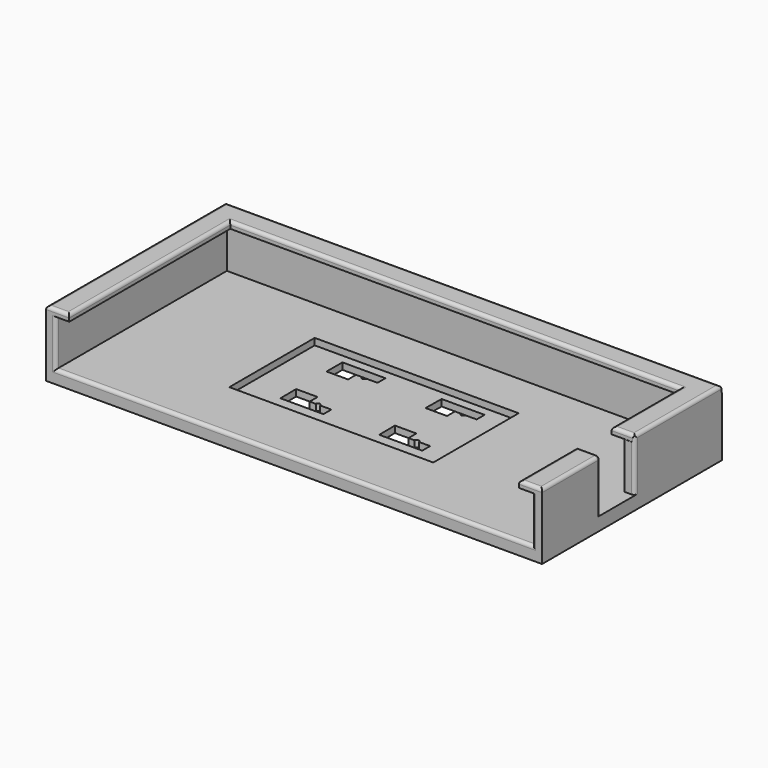
from build123d import *

# Parameters (mm, degrees)
F0_W         = 150
F0_H         = 68
F0_W_2       = 61.6867046999
F0_H_2       = 32.2795761846
F1_DEPTH     = 2
F2_W         = 3
F2_H         = 3.4045838118
F2_W_2       = 144
F2_H_2       = 64.5954161882
F2_H_3       = 29.5954161882
F2_H_4       = 22
F3_DEPTH     = 14
F4_W         = 4.8811412584
F4_H         = 7
F4_W_2       = 136
F4_W_3       = 7
F4_H_2       = 25.8289493918
F4_H_3       = 22
F5_DEPTH     = 2
F6_T1_DEPTH  = 72.8877383471
F6_T3_DEPTH  = 12
F6_T5_DEPTH  = 63.3877383471
F6_T7_DEPTH  = 136
F6_T9_DEPTH  = 28.3289493918
F6_T11_DEPTH = 12
F6_T13_DEPTH = 37.8289493918
F6_T15_DEPTH = 155
F6_T17_DEPTH = 23.5
F6_T19_DEPTH = 8.5
F6_T21_DEPTH = 27
F6_T23_DEPTH = 144
F6_T25_DEPTH = 14
F6_T27_DEPTH = 15
F6_T29_DEPTH = 16.5
F6_S33_W     = 1
F6_S33_H     = 1
F6_T34_DEPTH = 1
F6_T41_DEPTH = 65.8877383471
F6_T45_DEPTH = 138.5
F6_T52_DEPTH = 138.5
F6_T56_DEPTH = 30.8289493918
F6_T63_DEPTH = 146.5
F6_T67_DEPTH = 16.5
F6_T74_DEPTH = 146.5
F6_T78_DEPTH = 16.5
F7_W         = 150
F7_H         = 68
F7_W_2       = 61.6867046999
F7_H_2       = 32.2795761846
F8_DEPTH     = 2
F9_W         = 73.8973718075
F9_H         = 39.0960725045
F9_W_2       = 61.6867046999
F9_H_2       = 32.2795761846
F10_DEPTH    = 2


# Not quite as in the source:
# - a fillet or chamfer that OpenCascade refuses, or shapes differently, is made with other operations: its cross-section is extruded or revolved along the edge and cut away or added
# - a feature names something its author has since deleted; it is built from what else it names


with BuildPart() as f1:
    # F0 (on Top) → F1 (new body)
    with BuildSketch(Plane.XY):
        with Locations((75, 34)):
            Rectangle(F0_W, F0_H)
        with Locations((71.4499814534, 34.6545311671)):
            Rectangle(F0_W_2, F0_H_2, mode=Mode.SUBTRACT)
    extrude(amount=F1_DEPTH)

    # F2 (on face) → F3 (join)
    with BuildSketch(Plane.XY.offset(2)):
        with Locations((1.5, 66.2977080941)):
            Rectangle(F2_W, F2_H)
        with Locations((75, 66.2977080941)):
            Rectangle(F2_W_2, F2_H)
        with Locations((1.5, 32.2977080941)):
            Rectangle(F2_W, F2_H_2)
        with Locations((148.5, 66.2977080941)):
            Rectangle(F2_W, F2_H)
        with Locations((148.5, 49.7977080941)):
            Rectangle(F2_W, F2_H_3)
        with Locations((148.5, 11)):
            Rectangle(F2_W, F2_H_4)
    extrude(amount=F3_DEPTH)

    # F4 (on face) → F5 (join)
    with BuildSketch(Plane.XY.offset(16)):
        Polygon((0, 67.8877383471), (0, 0), (7, 0), (7, 60.8877383471), (2.1188587416, 60.8877383471), (2.1188587416, 67.8877383471), align=None)
        with Locations((4.5594293708, 64.3877383471)):
            Rectangle(F4_W, F4_H)
        with Locations((75, 64.3877383471)):
            Rectangle(F4_W_2, F4_H)
        with Locations((146.5, 64.3877383471)):
            Rectangle(F4_W_3, F4_H)
        with Locations((146.5, 47.9732636511)):
            Rectangle(F4_W_3, F4_H_2)
        with Locations((146.5, 11)):
            Rectangle(F4_W_3, F4_H_3)
    extrude(amount=F5_DEPTH)

    # F6: fillet of radius 1 on 17 edges, made by hand

    # F6_s2 → F6_t1 (cut)
    with BuildSketch(Plane.XZ.offset(-70.3877383471)):
        with BuildLine():
            ThreePointArc((0, 17), (0.2928932188, 17.7071067812), (1, 18))
            Line((1, 18), (0, 18))
            Line((0, 18), (0, 17))
        make_face()
    extrude(amount=F6_T1_DEPTH, mode=Mode.SUBTRACT)

    # F6_s4 → F6_t3 (cut)
    with BuildSketch(Plane.YZ.offset(-2.5)):
        with BuildLine():
            ThreePointArc((0, 17), (0.2928932188, 17.7071067812), (1, 18))
            Line((1, 18), (0, 18))
            Line((0, 18), (0, 17))
        make_face()
    extrude(amount=F6_T3_DEPTH, mode=Mode.SUBTRACT)

    # F6_s6 → F6_t5 (cut)
    with BuildSketch(Plane.XZ.offset(-60.8877383471)):
        with BuildLine():
            ThreePointArc((7, 17), (6.7071067812, 17.7071067812), (6, 18))
            Line((6, 18), (7, 18))
            Line((7, 18), (7, 17))
        make_face()
    extrude(amount=F6_T5_DEPTH, mode=Mode.SUBTRACT)

    # F6_s8 → F6_t7 (cut)
    with BuildSketch(Plane.YZ.offset(7)):
        with BuildLine():
            ThreePointArc((60.8877383471, 17), (61.1806315659, 17.7071067812), (61.8877383471, 18))
            Line((61.8877383471, 18), (60.8877383471, 18))
            Line((60.8877383471, 18), (60.8877383471, 17))
        make_face()
    extrude(amount=F6_T7_DEPTH, mode=Mode.SUBTRACT)

    # F6_s10 → F6_t9 (cut)
    with BuildSketch(Plane.XZ.offset(-60.8877383471)):
        with BuildLine():
            ThreePointArc((143, 17), (143.2928932188, 17.7071067812), (144, 18))
            Line((144, 18), (143, 18))
            Line((143, 18), (143, 17))
        make_face()
    extrude(amount=F6_T9_DEPTH, mode=Mode.SUBTRACT)

    # F6_s12 → F6_t11 (cut)
    with BuildSketch(Plane.YZ.offset(140.5)):
        with BuildLine():
            ThreePointArc((35.0587889552, 17), (35.351682174, 17.7071067812), (36.0587889552, 18))
            Line((36.0587889552, 18), (35.0587889552, 18))
            Line((35.0587889552, 18), (35.0587889552, 17))
        make_face()
        with BuildLine():
            ThreePointArc((1, 18), (0.2928932188, 17.7071067812), (0, 17))
            Line((0, 17), (0, 18))
            Line((0, 18), (1, 18))
        make_face()
    extrude(amount=F6_T11_DEPTH, mode=Mode.SUBTRACT)

    # F6_s14 → F6_t13 (cut)
    with BuildSketch(Plane.XZ.offset(-70.3877383471)):
        with BuildLine():
            ThreePointArc((150, 17), (149.7071067812, 17.7071067812), (149, 18))
            Line((149, 18), (150, 18))
            Line((150, 18), (150, 17))
        make_face()
    extrude(amount=F6_T13_DEPTH, mode=Mode.SUBTRACT)

    # F6_s16 → F6_t15 (cut)
    with BuildSketch(Plane.YZ.offset(-2.5)):
        with BuildLine():
            ThreePointArc((66.8877383471, 18), (67.5948451282, 17.7071067812), (67.8877383471, 17))
            Line((67.8877383471, 17), (67.8877383471, 18))
            Line((67.8877383471, 18), (66.8877383471, 18))
        make_face()
    extrude(amount=F6_T15_DEPTH, mode=Mode.SUBTRACT)

    # F6_s18 → F6_t17 (cut)
    with BuildSketch(Plane.XZ.offset(-21)):
        with BuildLine():
            ThreePointArc((149, 18), (149.7071067812, 17.7071067812), (150, 17))
            Line((150, 17), (150, 18))
            Line((150, 18), (149, 18))
        make_face()
    extrude(amount=F6_T17_DEPTH, mode=Mode.SUBTRACT)

    # F6_s20 → F6_t19 (cut)
    with BuildSketch(Plane.YZ.offset(140.5)):
        with BuildLine():
            ThreePointArc((21, 18), (21.7071067812, 17.7071067812), (22, 17))
            Line((22, 17), (22, 18))
            Line((22, 18), (21, 18))
        make_face()
    extrude(amount=F6_T19_DEPTH, mode=Mode.SUBTRACT)

    # F6_s22 → F6_t21 (cut)
    with BuildSketch(Plane.XZ.offset(-24.5)):
        with BuildLine():
            ThreePointArc((143, 17), (143.2928932188, 17.7071067812), (144, 18))
            Line((144, 18), (143, 18))
            Line((143, 18), (143, 17))
        make_face()
    extrude(amount=F6_T21_DEPTH, mode=Mode.SUBTRACT)

    # F6_s24 → F6_t23 (cut)
    with BuildSketch(Plane.YZ.offset(3)):
        with BuildLine():
            ThreePointArc((1, 2), (0.2928932188, 1.7071067812), (0, 1))
            Line((0, 1), (0, 2))
            Line((0, 2), (1, 2))
        make_face()
    extrude(amount=F6_T23_DEPTH, mode=Mode.SUBTRACT)

    # F6_s26 → F6_t25 (cut)
    with BuildSketch(Plane.XY.offset(2)):
        with BuildLine():
            ThreePointArc((3, 1), (2.7071067812, 0.2928932188), (2, 0))
            Line((2, 0), (3, 0))
            Line((3, 0), (3, 1))
        make_face()
        with BuildLine():
            ThreePointArc((147, 1), (147.2928932188, 0.2928932188), (148, 0))
            Line((148, 0), (147, 0))
            Line((147, 0), (147, 1))
        make_face()
    extrude(amount=F6_T25_DEPTH, mode=Mode.SUBTRACT)

    # F6_s28 → F6_t27 (cut)
    with BuildSketch(Plane.XY.offset(2)):
        with BuildLine():
            ThreePointArc((149, 22), (149.7071067812, 21.7071067812), (150, 21))
            Line((150, 21), (150, 22))
            Line((150, 22), (149, 22))
        make_face()
    extrude(amount=F6_T27_DEPTH, mode=Mode.SUBTRACT)

    # F6_s30 → F6_t29 (cut)
    with BuildSketch(Plane.XY.offset(2)):
        with BuildLine():
            ThreePointArc((149, 35), (149.7071067812, 35.2928932188), (150, 36))
            Line((150, 36), (150, 35))
            Line((150, 35), (149, 35))
        make_face()
    extrude(amount=F6_T29_DEPTH, mode=Mode.SUBTRACT)


with BuildPart() as f6_tool32:
    # F6_s33 → F6_t34 (new body)
    with BuildSketch(Plane.XZ.offset(-21)):
        with Locations((149.5, 17.5)):
            Rectangle(F6_S33_W, F6_S33_H)
    extrude(amount=-F6_T34_DEPTH)

    # F6_s35 → F6_t36 (revolve, cut)
    with BuildSketch(Plane(origin=(149, 21, 17), x_dir=(-0.7071067812, 0, -0.7071067812), z_dir=(0.7071067812, 0, -0.7071067812))):
        with BuildLine():
            ThreePointArc((0, -1), (1, 0), (0, 1))
            Line((0, 1), (0, -1))
        make_face()
    revolve(axis=Axis((149, 21, 17), (0, 1, 0)), mode=Mode.SUBTRACT)


with BuildPart() as f1_1:
    add(f1.part)

    # F6_t31: cut F6_tool32
    add(f6_tool32.part, mode=Mode.SUBTRACT)


with BuildPart() as f6_tool39:
    # F6_s40 → F6_t41 (new body)
    with BuildSketch(Plane.XZ.offset(2.5)):
        with BuildLine():
            ThreePointArc((7, 17), (6.7071067812, 17.7071067812), (6, 18))
            Line((6, 18), (7, 18))
            Line((7, 18), (7, 17))
        make_face()
    extrude(amount=-F6_T41_DEPTH)

    split(bisect_by=Plane.XZ.offset(-60.8877383471), keep=Keep.BOTTOM)


with BuildPart() as f6_tool43:
    # F6_s44 → F6_t45 (new body)
    with BuildSketch(Plane.YZ.offset(4.5)):
        with BuildLine():
            ThreePointArc((60.8877383471, 17), (61.1806315659, 17.7071067812), (61.8877383471, 18))
            Line((61.8877383471, 18), (60.8877383471, 18))
            Line((60.8877383471, 18), (60.8877383471, 17))
        make_face()
    extrude(amount=F6_T45_DEPTH)

    split(bisect_by=Plane.YZ.offset(7), keep=Keep.BOTTOM)


with BuildPart() as f6_tool39_1:
    add(f6_tool39.part)

    # F6_t47: intersect F6_tool43
    add(f6_tool43.part, mode=Mode.INTERSECT)


with BuildPart() as f1_2:
    add(f1_1.part)

    # F6_t37: cut F6_tool39
    add(f6_tool39_1.part, mode=Mode.SUBTRACT)


with BuildPart() as f6_tool50:
    # F6_s51 → F6_t52 (new body)
    with BuildSketch(Plane.YZ.offset(7)):
        with BuildLine():
            ThreePointArc((60.8877383471, 17), (61.1806315659, 17.7071067812), (61.8877383471, 18))
            Line((61.8877383471, 18), (60.8877383471, 18))
            Line((60.8877383471, 18), (60.8877383471, 17))
        make_face()
    extrude(amount=F6_T52_DEPTH)

    split(bisect_by=Plane.YZ.offset(143), keep=Keep.TOP)


with BuildPart() as f6_tool54:
    # F6_s55 → F6_t56 (new body)
    with BuildSketch(Plane.XZ.offset(-63.3877383471)):
        with BuildLine():
            ThreePointArc((143, 17), (143.2928932188, 17.7071067812), (144, 18))
            Line((144, 18), (143, 18))
            Line((143, 18), (143, 17))
        make_face()
    extrude(amount=F6_T56_DEPTH)

    split(bisect_by=Plane.XZ.offset(-60.8877383471), keep=Keep.BOTTOM)


with BuildPart() as f6_tool50_1:
    add(f6_tool50.part)

    # F6_t58: intersect F6_tool54
    add(f6_tool54.part, mode=Mode.INTERSECT)


with BuildPart() as f1_3:
    add(f1_2.part)

    # F6_t48: cut F6_tool50
    add(f6_tool50_1.part, mode=Mode.SUBTRACT)


with BuildPart() as f6_tool61:
    # F6_s62 → F6_t63 (new body)
    with BuildSketch(Plane.YZ.offset(0.5)):
        with BuildLine():
            ThreePointArc((1, 2), (0.2928932188, 1.7071067812), (0, 1))
            Line((0, 1), (0, 2))
            Line((0, 2), (1, 2))
        make_face()
    extrude(amount=F6_T63_DEPTH)

    split(bisect_by=Plane.YZ.offset(3), keep=Keep.BOTTOM)


with BuildPart() as f6_tool65:
    # F6_s66 → F6_t67 (new body)
    with BuildSketch(Plane.XY.offset(-0.5)):
        with BuildLine():
            ThreePointArc((3, 1), (2.7071067812, 0.2928932188), (2, 0))
            Line((2, 0), (3, 0))
            Line((3, 0), (3, 1))
        make_face()
    extrude(amount=F6_T67_DEPTH)

    split(bisect_by=Plane.XY.offset(2), keep=Keep.BOTTOM)


with BuildPart() as f6_tool61_1:
    add(f6_tool61.part)

    # F6_t69: intersect F6_tool65
    add(f6_tool65.part, mode=Mode.INTERSECT)


with BuildPart() as f1_4:
    add(f1_3.part)

    # F6_t59: cut F6_tool61
    add(f6_tool61_1.part, mode=Mode.SUBTRACT)


with BuildPart() as f6_tool72:
    # F6_s73 → F6_t74 (new body)
    with BuildSketch(Plane.YZ.offset(3)):
        with BuildLine():
            ThreePointArc((1, 2), (0.2928932188, 1.7071067812), (0, 1))
            Line((0, 1), (0, 2))
            Line((0, 2), (1, 2))
        make_face()
    extrude(amount=F6_T74_DEPTH)

    split(bisect_by=Plane.YZ.offset(147), keep=Keep.TOP)


with BuildPart() as f6_tool76:
    # F6_s77 → F6_t78 (new body)
    with BuildSketch(Plane.XY.offset(-0.5)):
        with BuildLine():
            ThreePointArc((147, 1), (147.2928932188, 0.2928932188), (148, 0))
            Line((148, 0), (147, 0))
            Line((147, 0), (147, 1))
        make_face()
    extrude(amount=F6_T78_DEPTH)

    split(bisect_by=Plane.XY.offset(2), keep=Keep.BOTTOM)


with BuildPart() as f6_tool72_1:
    add(f6_tool72.part)

    # F6_t80: intersect F6_tool76
    add(f6_tool76.part, mode=Mode.INTERSECT)


with BuildPart() as f1_5:
    add(f1_4.part)

    # F6_t70: cut F6_tool72
    add(f6_tool72_1.part, mode=Mode.SUBTRACT)

    # F7 (on face) → F8 (join)
    with BuildSketch(Plane.XY):
        with Locations((75, 34)):
            Rectangle(F7_W, F7_H)
        with Locations((71.4499814534, 34.6545311671)):
            Rectangle(F7_W_2, F7_H_2, mode=Mode.SUBTRACT)
    extrude(amount=-F8_DEPTH)

    # F9 (on face) → F10 (join)
    with BuildSketch(Plane.XY):
        with Locations((72.7380400409, 34.5662031323)):
            Rectangle(F9_W, F9_H)
        with Locations((71.4499814534, 34.6545311671)):
            Rectangle(F9_W_2, F9_H_2, mode=Mode.SUBTRACT)
        with Locations((71.4499814534, 34.6545311671)):
            Rectangle(F9_W_2, F9_H_2)
        with BuildLine():
            Line((64.1806087643, 24.6144512218), (51.1806087643, 24.6144512218))
            Line((51.1806087643, 24.6144512218), (51.1301904917, 30.6142393845))
            Line((51.1301904917, 30.6142393845), (57.6295237077, 30.6142393845))
            Line((57.6295237077, 30.6142393845), (57.6295237077, 27.6144512218))
            Line((57.6295237077, 27.6144512218), (59.4795237077, 27.6144512218))
            ThreePointArc((59.4795237077, 27.6144512218), (60.1295237077, 28.2644512218), (60.7795237077, 27.6144512218))
            Line((60.7795237077, 27.6144512218), (64.1806087643, 27.6144512218))
            Line((64.1806087643, 27.6144512218), (64.1806087643, 24.6144512218))
        make_face(mode=Mode.SUBTRACT)
        with BuildLine():
            Line((94.0630321503, 24.6144512218), (81.0630321503, 24.6144512218))
            Line((81.0630321503, 24.6144512218), (81.0126138777, 30.6142393845))
            Line((81.0126138777, 30.6142393845), (87.5119470937, 30.6142393845))
            Line((87.5119470937, 30.6142393845), (87.5119470937, 27.6144512218))
            Line((87.5119470937, 27.6144512218), (89.3619470937, 27.6144512218))
            ThreePointArc((89.3619470937, 27.6144512218), (90.0119470937, 28.2644512218), (90.6619470937, 27.6144512218))
            Line((90.6619470937, 27.6144512218), (94.0630321503, 27.6144512218))
            Line((94.0630321503, 27.6144512218), (94.0630321503, 24.6144512218))
        make_face(mode=Mode.SUBTRACT)
        with BuildLine():
            Line((51.1387947655, 42.1142393845), (51.1387947655, 48.1142393845))
            Line((51.1387947655, 48.1142393845), (64.1387947655, 48.1142393845))
            Line((64.1387947655, 48.1142393845), (64.1387947655, 45.1142393845))
            Line((64.1387947655, 45.1142393845), (60.7887947655, 45.1142393845))
            ThreePointArc((60.7887947655, 45.1142393845), (60.1387947655, 44.4642393845), (59.4887947655, 45.1142393845))
            Line((59.4887947655, 45.1142393845), (57.6387947655, 45.1142393845))
            Line((57.6387947655, 45.1142393845), (57.6387947655, 42.1142393845))
            Line((57.6387947655, 42.1142393845), (51.1387947655, 42.1142393845))
        make_face(mode=Mode.SUBTRACT)
        with BuildLine():
            Line((81.063032589, 42.1147177292), (81.1387947655, 48.1142393845))
            Line((81.1387947655, 48.1142393845), (94.1387947655, 48.1142393845))
            Line((94.1387947655, 48.1142393845), (94.1387947655, 45.1142393845))
            Line((94.1387947655, 45.1142393845), (90.713032589, 45.1142393845))
            ThreePointArc((90.713032589, 45.1142393845), (90.063032589, 44.4642393845), (89.413032589, 45.1142393845))
            Line((89.413032589, 45.1142393845), (87.563032589, 45.1142393845))
            Line((87.563032589, 45.1142393845), (87.563032589, 42.1147177292))
            Line((87.563032589, 42.1147177292), (81.063032589, 42.1147177292))
        make_face(mode=Mode.SUBTRACT)
    extrude(amount=-F10_DEPTH)


solid = f1_5.part
